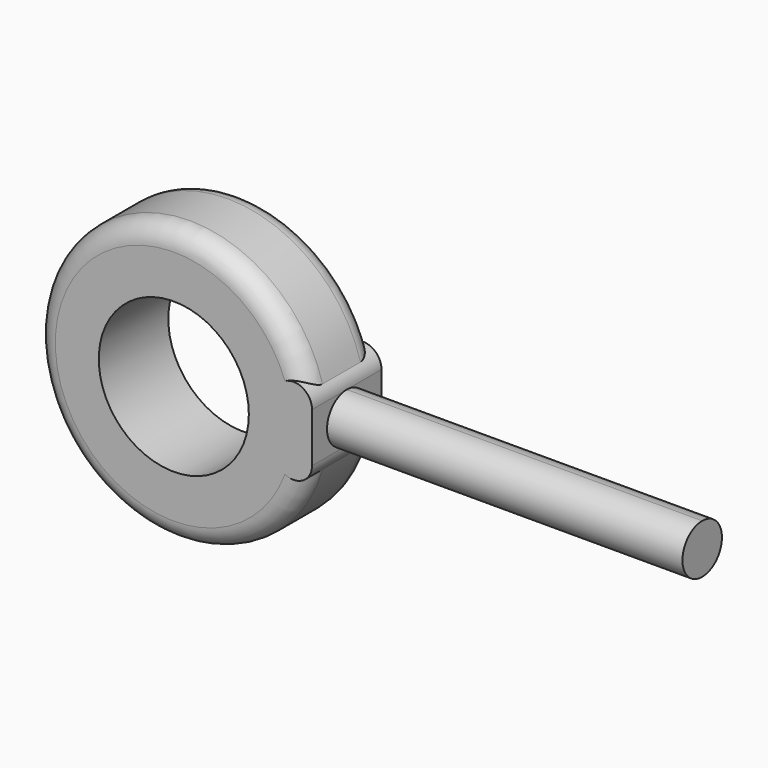
from build123d import *

# Parameters (mm, degrees)
F0_R     = 4.826
F1_DEPTH = 5.588
F3_DEPTH = 22.86
F4_R     = 1.27
F5_R     = 1.27


# Not quite as in the source:
# - a feature names something its author has since deleted; it is built from what else it names


with BuildPart() as f1:
    # F0 (on Front) → F1 (new body)
    with BuildSketch(Plane.XZ):
        with BuildLine():
            Line((-22.86, -1.5875), (-22.86, 1.5875))
            ThreePointArc((-22.86, 1.5875), (-22.9466228701, 2.0329296457), (-23.1938651263, 2.4134324153))
            ThreePointArc((-23.1938651263, 2.4134324153), (-40.64, 0), (-23.1938651263, -2.4134324153))
            ThreePointArc((-23.1938651263, -2.4134324153), (-22.9466228701, -2.0329296457), (-22.86, -1.5875))
        make_face()
        with Locations((-31.75, 0)):
            Circle(F0_R, mode=Mode.SUBTRACT)
        Polygon((0, -1.5875), (0, 0), (0, 1.5875), (-22.86, 1.5875), (-22.86, -1.5875), align=None)
    extrude(amount=F1_DEPTH)

    # F2 (on face) → F3 (cut, through all)
    with BuildSketch(Plane.YZ):
        with BuildLine():
            ThreePointArc((-2.794, -1.5875), (-4.3815, 0), (-2.794, 1.5875))
            Line((-2.794, 1.5875), (-5.588, 1.5875))
            Line((-5.588, 1.5875), (-5.588, -1.5875))
            Line((-5.588, -1.5875), (-2.794, -1.5875))
        make_face()
        with BuildLine():
            ThreePointArc((-2.794, 1.5875), (-1.6714679849, 1.1225320151), (-1.2065, 0))
            ThreePointArc((-1.2065, 0), (-1.6714679849, -1.1225320151), (-2.794, -1.5875))
            Line((-2.794, -1.5875), (0, -1.5875))
            Line((0, -1.5875), (0, 1.5875))
            Line((0, 1.5875), (-2.794, 1.5875))
        make_face()
    extrude(amount=-F3_DEPTH, mode=Mode.SUBTRACT)

    # F4
    f4_edges = [f1.edges().sort_by_distance(p)[0] for p in [
        (-40.64, 0, 0),
    ]]
    fillet(f4_edges, radius=F4_R)

    # F5
    f5_edges = [f1.edges().sort_by_distance(p)[0] for p in [
        (-40.64, -5.588, 0),
    ]]
    fillet(f5_edges, radius=F5_R)


solid = f1.part
